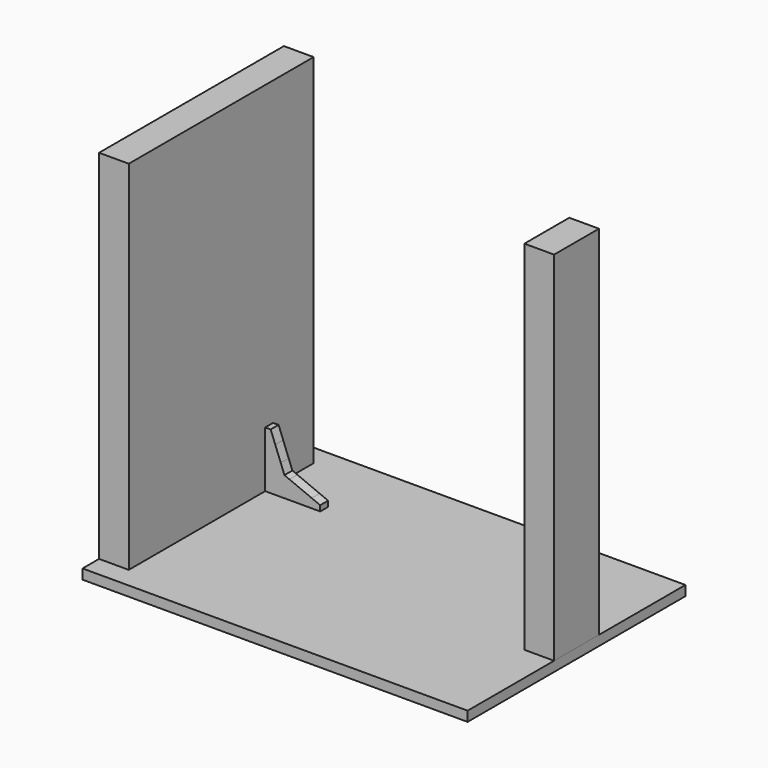
from build123d import *

# Parameters (mm, degrees)
F0_W      = 700
F0_H      = 495
F1_DEPTH  = 18
F2_W      = 54
F2_H      = 420
F3_DEPTH  = 650
F2_H_2    = 102
F4_W      = 102
F4_H      = 650
F5_DEPTH  = 700.001
F6_W      = 18
F6_H      = 102
F7_DEPTH  = 100
F8_DEPTH  = 650
F10_DEPTH = 25


# Not quite as in the source:
# - a feature names something its author has since deleted; it is built from what else it names


with BuildPart() as f1:
    # F0 (on Top) → F1 (new body)
    with BuildSketch(Plane.XY):
        Rectangle(F0_W, F0_H)
    extrude(amount=F1_DEPTH)


with BuildPart() as f3:
    # F2 (on face) → F3 (new body)
    with BuildSketch(Plane.XY.offset(18)):
        with Locations((-323, 0)):
            Rectangle(F2_W, F2_H)
    extrude(amount=F3_DEPTH)


with BuildPart() as f3b:
    # F2 (on face) → F3, piece 2 (new body)
    with BuildSketch(Plane.XY.offset(18)):
        with Locations((323, 0)):
            Rectangle(F2_W, F2_H_2)
    extrude(amount=F3_DEPTH)


with BuildPart() as f5_tool:
    # F4 (on face) → F5 (new body, through all)
    with BuildSketch(Plane.YZ.offset(350)):
        with Locations((0, 343)):
            Rectangle(F4_W, F4_H)
    extrude(amount=-F5_DEPTH)


with BuildPart() as f3_1:
    add(f3.part)

    # F5: cut by f5_tool
    add(f5_tool.part, mode=Mode.SUBTRACT)

    # F2 (on face) → F8 (join)
    with BuildSketch(Plane.XY.offset(18)):
        with Locations((-323, 0)):
            Rectangle(F2_W, F2_H)
    extrude(amount=F8_DEPTH)


with BuildPart() as f3b_1:
    add(f3b.part)

    # F5: cut by f5_tool
    add(f5_tool.part, mode=Mode.SUBTRACT)


with BuildPart() as f7:
    # F6 (on face) → F7 (new body)
    with BuildSketch(Plane.YZ.offset(-296)):
        with Locations((109, 69)):
            Rectangle(F6_W, F6_H)
    extrude(amount=F7_DEPTH)

    # F9 (on face) → F10 (cut)
    with BuildSketch(Plane(origin=(0, 118, 0), x_dir=(-1, 0, 0), z_dir=(0, 1, 0))):
        Polygon((261, 55), (267.7467766581, 72.5416193109), (277.7322773327, 98.5039210651), (286, 120), (251, 120), (196, 120), (196, 28), (211.3627376398, 34.3814448658), (251.799326006, 51.1781815717), align=None)
    extrude(amount=-F10_DEPTH, mode=Mode.SUBTRACT)


with BuildPart() as f8:
    # F2 (on face) → F8, piece 2 (new body)
    with BuildSketch(Plane.XY.offset(18)):
        with Locations((323, 0)):
            Rectangle(F2_W, F2_H_2)
    extrude(amount=F8_DEPTH)


solid = Compound([f1.part, f3_1.part, f7.part, f8.part])
